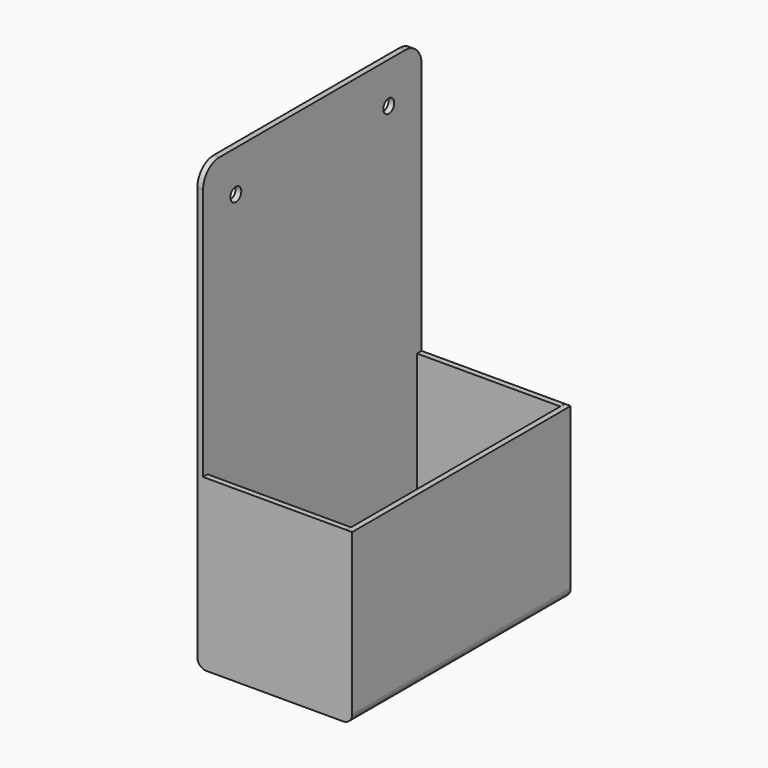
from build123d import *

# Parameters (mm, degrees)
F1_DEPTH    = 63.5
F3_DEPTH    = 2.667
F5_T4_DEPTH = 71.247
F6_T4_DEPTH = 71.247
F8_D        = 6.35
F9_R        = 9.525


# Not quite as in the source:
# - a fillet or chamfer that OpenCascade refuses, or shapes differently, is made with other operations: its cross-section is extruded or revolved along the edge and cut away or added
# - a feature of the source that left no trace in its solid (it failed there, or was rolled back) is left out


with BuildPart() as f1:
    # F0 (on Front) → F1 (new body, symmetric)
    with BuildSketch(Plane.XZ):
        with BuildLine():
            Line((65.151, 0), (1.524, 0))
            ThreePointArc((1.524, 0), (0.4463692655, 0.4463692655), (0, 1.524))
            Line((0, 1.524), (0, 76.2))
            Line((0, 76.2), (0, 203.2))
            Line((0, 203.2), (-2.667, 203.2))
            Line((-2.667, 203.2), (-2.667, 76.2))
            Line((-2.667, 76.2), (-2.667, 1.524))
            ThreePointArc((-2.667, 1.524), (-1.43948452, -1.43948452), (1.524, -2.667))
            Line((1.524, -2.667), (65.151, -2.667))
            ThreePointArc((65.151, -2.667), (68.11448452, -1.43948452), (69.342, 1.524))
            Line((69.342, 1.524), (69.342, 76.2))
            Line((69.342, 76.2), (66.675, 76.2))
            Line((66.675, 76.2), (66.675, 1.524))
            ThreePointArc((66.675, 1.524), (66.2286307345, 0.4463692655), (65.151, 0))
        make_face()
    extrude(amount=F1_DEPTH, both=True)

    # F2 (on face) → F3 (join)
    with BuildSketch(Plane.XZ.offset(63.5)):
        with BuildLine():
            Line((66.6496, -1.143), (66.6496, 76.2))
            Line((66.6496, 76.2), (0.0254, 76.2))
            Line((0.0254, 76.2), (0.0254, -1.143))
            ThreePointArc((0.0254, -1.143), (0.4717692655, -2.2206307345), (1.5494, -2.667))
            Line((1.5494, -2.667), (65.1256, -2.667))
            ThreePointArc((65.1256, -2.667), (66.2032307345, -2.2206307345), (66.6496, -1.143))
        make_face()
    extrude(amount=-F3_DEPTH)

    # F4: F1 across plane


with BuildPart() as f1_1:
    add(f1.part)
    add(f1.part.mirror(Plane.XZ))

    # F5: fillet of radius 1.524 on 1 edges, made by hand


with BuildPart() as f5_tool2:
    # F5_s3 → F5_t4 (new body)
    with BuildSketch(Plane.YZ.offset(-2.286)):
        with BuildLine():
            ThreePointArc((-59.309, 0), (-60.3866307345, 0.4463692655), (-60.833, 1.524))
            Line((-60.833, 1.524), (-60.833, 0))
            Line((-60.833, 0), (-59.309, 0))
        make_face()
    extrude(amount=F5_T4_DEPTH)

    split(bisect_by=Plane.YZ.offset(0.0254), keep=Keep.TOP)

    split(bisect_by=Plane.YZ.offset(66.6496), keep=Keep.BOTTOM)


with BuildPart() as f1_2:
    add(f1_1.part)

    # F5_t1: union F5_tool2
    add(f5_tool2.part)

    # F6: fillet of radius 1.524 on 1 edges, made by hand


with BuildPart() as f6_tool2:
    # F6_s3 → F6_t4 (new body)
    with BuildSketch(Plane.YZ.offset(-2.286)):
        with BuildLine():
            ThreePointArc((59.309, 0), (60.3866307345, 0.4463692655), (60.833, 1.524))
            Line((60.833, 1.524), (60.833, 0))
            Line((60.833, 0), (59.309, 0))
        make_face()
    extrude(amount=F6_T4_DEPTH)

    split(bisect_by=Plane.YZ.offset(0.0254), keep=Keep.TOP)

    split(bisect_by=Plane.YZ.offset(66.6496), keep=Keep.BOTTOM)


with BuildPart() as f1_3:
    add(f1_2.part)

    # F6_t1: union F6_tool2
    add(f6_tool2.part)

    # F8 (through all)
    with Locations(Plane.YZ):
        with Locations((-44.45, 184.15), (44.45, 184.15)):
            Hole(F8_D / 2)

    # F9
    f9_edges = [f1_3.edges().sort_by_distance(p)[0] for p in [
        (-1.3335, -63.5, 203.2),
        (-1.3335, 63.5, 203.2),
    ]]
    fillet(f9_edges, radius=F9_R)


solid = f1_3.part
